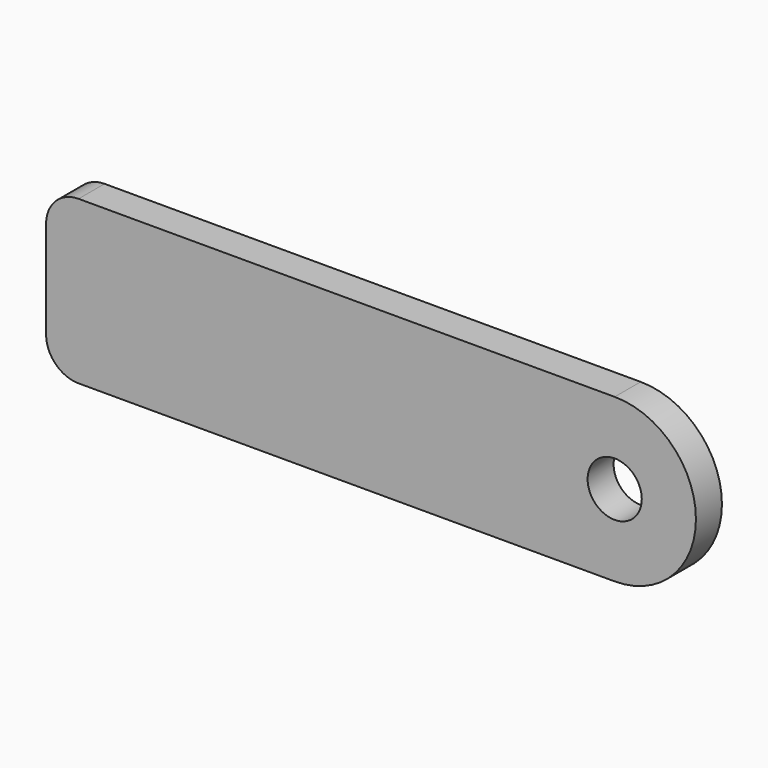
from build123d import *

# Parameters (mm, degrees)
F0_R         = 2.5
F1_DEPTH     = 3
F2_TEXT_SIZE = 8.9020771513
F3_DEPTH     = 1
F5_DEPTH     = 1


# Not quite as in the source:
# - Text() gives the source's letters only with a copy of the font that has no kerning and outlines rounded to 1/6400 em; it was checked with that copy


with BuildPart() as f1:
    # F0 (on Front) → F1 (new body)
    with BuildSketch(Plane.XZ):
        with BuildLine():
            Line((52.5, 15), (3, 15))
            ThreePointArc((3, 15), (0.8786796564, 14.1213203436), (0, 12))
            Line((0, 12), (0, 3))
            ThreePointArc((0, 3), (0.8786796564, 0.8786796564), (3, 0))
            Line((3, 0), (52.5, 0))
            ThreePointArc((52.5, 0), (60, 7.5), (52.5, 15))
        make_face()
        with Locations((52.5, 7.5)):
            Circle(F0_R, mode=Mode.SUBTRACT)
    extrude(amount=-F1_DEPTH)

    # F2 (on face) → F3 (join)
    with BuildSketch(Plane(origin=(0, 3, 0), x_dir=(-1, 0, 0), z_dir=(0, 1, 0))):
        with Locations((-35, 4.2952522255)):
            Text('samuel', F2_TEXT_SIZE, font='Open Sans', text_align=(TextAlign.LEFT, TextAlign.BOTTOM))
    extrude(amount=F3_DEPTH)

    # F4 (on face) → F5 (cut)
    with BuildSketch(Plane(origin=(0, 3, 0), x_dir=(-1, 0, 0), z_dir=(0, 1, 0))):
        with BuildLine():
            ThreePointArc((-1.5, 12), (-1.9393398282, 13.0606601718), (-3, 13.5))
            Line((-3, 13.5), (-52.5, 13.5))
            ThreePointArc((-52.5, 13.5), (-58.5, 7.5), (-52.5, 1.5))
            Line((-52.5, 1.5), (-3, 1.5))
            ThreePointArc((-3, 1.5), (-1.9393398282, 1.9393398282), (-1.5, 3))
            Line((-1.5, 3), (-1.5, 12))
        make_face()
        with BuildLine():
            Line((-52.5, 13), (-3, 13))
            ThreePointArc((-3, 13), (-2.2928932188, 12.7071067812), (-2, 12))
            Line((-2, 12), (-2, 3))
            ThreePointArc((-2, 3), (-2.2928932188, 2.2928932188), (-3, 2))
            Line((-3, 2), (-52.5, 2))
            ThreePointArc((-52.5, 2), (-58, 7.5), (-52.5, 13))
        make_face(mode=Mode.SUBTRACT)
    extrude(amount=-F5_DEPTH, mode=Mode.SUBTRACT)


solid = f1.part
